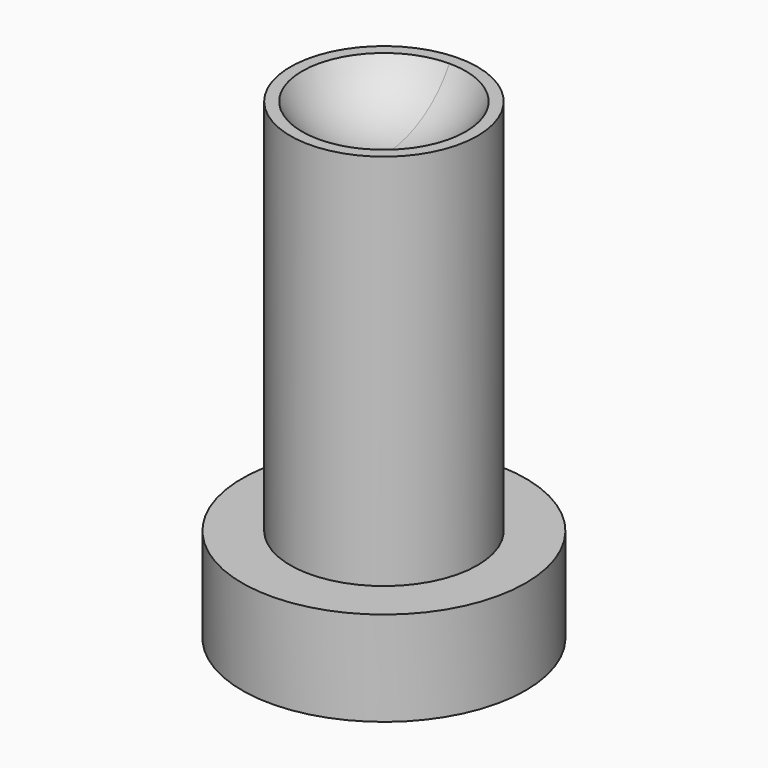
from build123d import *
from build123d import SkipClean  # not in build123d's __all__

# Parameters (mm, degrees)
F0_R     = 19.05
F1_DEPTH = 12.7
F2_R     = 12.573
F3_DEPTH = 63.5


with BuildPart() as f1:
    # F0 (on Top) → F1 (new body)
    with BuildSketch(Plane.XY):
        Circle(F0_R)
    extrude(amount=F1_DEPTH)

    # F2 (on Top) → F3 (join)
    with BuildSketch(Plane.XY):
        Circle(F2_R)
    extrude(amount=F3_DEPTH)

    # F4 (on Right) → F6 (revolve, cut)
    with BuildSketch(Plane.YZ):
        with BuildLine():
            Line((12.7, 69.85), (-12.7, 69.85))
            ThreePointArc((-12.7, 69.85), (0, 57.15), (12.7, 69.85))
        make_face()
    with SkipClean():  # cleaning this boolean's faces spoils the solid; the shape is the same uncleaned
        revolve(axis=Axis((0, -1.6116397455, 69.85), (0, 1, 0)), mode=Mode.SUBTRACT)


solid = f1.part
